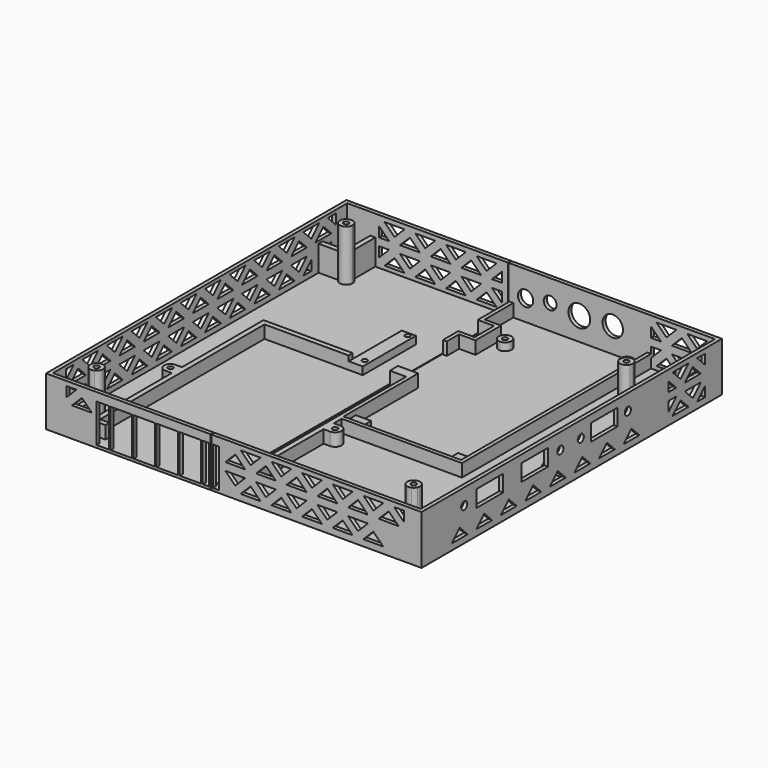
from build123d import *

# Parameters (mm, degrees)
F1_W           = 186.5100009048
F1_H           = 186.5100009048
F1_W_2         = 182.7000009048
F1_H_2         = 182.7000009048
F2_DEPTH       = 86.36
F5_W           = 186.5100009048
F5_H           = 186.5100009048
F6_DEPTH       = 1.27
F7_W           = 7.62
F7_H           = 7.62
F7_R           = 3.175
F7_R_2         = 1.27
F7_W_2         = 6.985
F7_H_2         = 33.02
F8_DEPTH       = 3.81
F9_R           = 1.27
F10_DEPTH      = 6.35
F11_R          = 5.08
F11_R_2        = 5.3975
F11_R_3        = 3.175
F11_R_4        = 3.81
F12_DEPTH      = 1.905
F13_W          = 10.668
F13_H          = 19.05
F14_DEPTH      = 2.54
F15_W          = 16.51
F15_H          = 8.255
F15_R          = 1.905
F16_DEPTH      = 1.905
F20_DEPTH      = 0.9525
F21_R          = 1.27
F22_DEPTH      = 12.7
F23_DEPTH      = 25.4
F24_W          = 8.763
F24_H          = 45.085
F24_W_2        = 11.938
F24_W_3        = 10.16
F25_DEPTH      = 25.4
F27_DEPTH      = 1.905
F29_DEPTH      = 2.54
F31_DEPTH      = 2.54
F33_DEPTH      = 2.54
F35_W          = 182.7000009048
F35_H          = 182.7000009048
F36_DEPTH      = 3.81
F37_DEPTH      = 25.4
F37_TAPER      = 45
F38_W          = 186.5100009048
F38_H          = 63.1952
F39_DEPTH      = 7.366
F41_DEPTH      = 179.1450009048
F42_W          = 5.715
F42_H          = 63.1952
F43_DEPTH      = 184.6060009048
F44_W          = 0.381
F44_H          = 186.5100009048
F45_DEPTH      = 1.271
F45_DEPTH_BACK = 25.401
F46_W          = 0.762
F46_H          = 1.905
F47_DEPTH      = 23.1648


with BuildPart() as f2:
    # F1 (on Top) → F2 (new body)
    with BuildSketch(Plane.XY):
        with Locations((78.65, -74.84)):
            Rectangle(F1_W, F1_H)
        with Locations((78.65, -74.84)):
            Rectangle(F1_W_2, F1_H_2, mode=Mode.SUBTRACT)
    extrude(amount=F2_DEPTH)

    # F5 (on Top) → F6 (join)
    with BuildSketch(Plane.XY):
        with Locations((78.65, -74.84)):
            Rectangle(F5_W, F5_H)
    extrude(amount=-F6_DEPTH)

    # F7 (on Top) → F8 (join)
    with BuildSketch(Plane.XY):
        with Locations((81.7350004524, -95.2499995476)):
            Rectangle(F7_W, F7_H)
        with Locations((132.5350004524, -95.2499995476)):
            Rectangle(F7_W, F7_H)
        with Locations((83.0050004524, -5.0799995476)):
            Circle(F7_R)
        with Locations((83.0050004524, -5.0799995476)):
            Circle(F7_R_2, mode=Mode.SUBTRACT)
        with Locations((131.2650004524, 10.1600004524)):
            Circle(F7_R)
        with Locations((131.2650004524, 10.1600004524)):
            Circle(F7_R_2, mode=Mode.SUBTRACT)
        with Locations((50.9375004524, -41.2749995476)):
            Rectangle(F7_W_2, F7_H_2)
        with Locations((51.8900004524, -53.3399995476)):
            Circle(F7_R_2, mode=Mode.SUBTRACT)
        with Locations((51.8900004524, -26.6699995476)):
            Circle(F7_R_2, mode=Mode.SUBTRACT)
    extrude(amount=F8_DEPTH)

    # F9 (on Top) → F10 (join)
    with BuildSketch(Plane.XY):
        Polygon((76.0200004524, -15.2399995476), (67.8920004524, -15.2399995476), (67.8920004524, -24.7649995476), (69.7970004524, -24.7649995476), (69.7970004524, -17.1449995476), (77.9250004524, -17.1449995476), (77.9250004524, -1.2699995476), (69.7970004524, -1.2699995476), (69.7970004524, 16.5100004524), (67.8920004524, 16.5100004524), (67.8920004524, -3.1749995476), (76.0200004524, -3.1749995476), align=None)
        with BuildLine():
            Line((136.3450004524, 16.5100004524), (136.3450004524, -99.0599995476))
            Line((136.3450004524, -99.0599995476), (77.9250004524, -99.0599995476))
            Line((77.9250004524, -99.0599995476), (77.9250004524, -52.7049995476))
            Line((77.9250004524, -52.7049995476), (67.8920004524, -52.7049995476))
            Line((67.8920004524, -52.7049995476), (67.8920004524, -57.7849995476))
            Line((67.8920004524, -57.7849995476), (76.0200004524, -57.7849995476))
            Line((76.0200004524, -57.7849995476), (76.0200004524, -100.9649995476))
            Line((76.0200004524, -100.9649995476), (76.0200004524, -159.84))
            Line((76.0200004524, -159.84), (71.3210004524, -159.84))
            Line((71.3210004524, -159.84), (71.3210004524, -162.38))
            Line((71.3210004524, -162.38), (78.5600004524, -162.38))
            Line((78.5600004524, -162.38), (78.5600004524, -112.215))
            Line((78.5600004524, -112.215), (81.7350004524, -112.215))
            ThreePointArc((81.7350004524, -112.215), (84.9100004524, -109.04), (81.7350004524, -105.865))
            Line((81.7350004524, -105.865), (78.5600004524, -105.865))
            Line((78.5600004524, -105.865), (78.5600004524, -100.9649995476))
            Line((78.5600004524, -100.9649995476), (138.2500004524, -100.9649995476))
            Line((138.2500004524, -100.9649995476), (138.2500004524, 16.5100004524))
            Line((138.2500004524, 16.5100004524), (136.3450004524, 16.5100004524))
        make_face()
        with Locations((81.7350004524, -109.04)):
            Circle(F9_R, mode=Mode.SUBTRACT)
        with BuildLine():
            Line((5.6620004524, -57.7849995476), (47.4450004524, -57.7849995476))
            Line((47.4450004524, -57.7849995476), (47.4450004524, -55.2449995476))
            Line((47.4450004524, -55.2449995476), (3.1220004524, -55.2449995476))
            Line((3.1220004524, -55.2449995476), (3.1220004524, -105.865))
            Line((3.1220004524, -105.865), (-0.0529995476, -105.865))
            ThreePointArc((-0.0529995476, -105.865), (-3.2279995476, -109.04), (-0.0529995476, -112.215))
            Line((-0.0529995476, -112.215), (3.1220004524, -112.215))
            Line((3.1220004524, -112.215), (3.1220004524, -162.38))
            Line((3.1220004524, -162.38), (10.3610004524, -162.38))
            Line((10.3610004524, -162.38), (10.3610004524, -159.84))
            Line((10.3610004524, -159.84), (5.6620004524, -159.84))
            Line((5.6620004524, -159.84), (5.6620004524, -57.7849995476))
        make_face()
        with Locations((-0.0529995476, -109.04)):
            Circle(F9_R, mode=Mode.SUBTRACT)
    extrude(amount=F10_DEPTH)

    # F11 (on face) → F12 (cut, through all)
    with BuildSketch(Plane(origin=(0, 18.4150004524, 0), x_dir=(-1, 0, 0), z_dir=(0, 1, 0))):
        with Locations((-119.2000004524, 12.319)):
            Circle(F11_R)
        with Locations((-102.5630004524, 11.43)):
            Circle(F11_R_2)
        with Locations((-88.0850004524, 12.319)):
            Circle(F11_R_3)
        with Locations((-75.8930004524, 10.414)):
            Circle(F11_R_4)
    extrude(amount=-F12_DEPTH, mode=Mode.SUBTRACT)

    # F13 (on face) → F14 (cut)
    with BuildSketch(Plane(origin=(0, -166.1900004524, 0), x_dir=(-1, 0, 0), z_dir=(0, 1, 0))):
        Polygon((-10.3610004524, 0), (-10.3610004524, 6.35), (-10.3610004524, 19.05), (-16.7110004524, 19.05), (-16.7110004524, 0), align=None)
        with Locations((-22.8070004524, 9.525)):
            Rectangle(F13_W, F13_H)
        with Locations((-34.2370004524, 9.525)):
            Rectangle(F13_W, F13_H)
        with Locations((-45.6670004524, 9.525)):
            Rectangle(F13_W, F13_H)
        with Locations((-57.0970004524, 9.525)):
            Rectangle(F13_W, F13_H)
        Polygon((-71.3210004524, 6.35), (-71.3210004524, 0), (-63.1930004524, 0), (-63.1930004524, 19.05), (-71.3210004524, 19.05), align=None)
    extrude(amount=-F14_DEPTH, mode=Mode.SUBTRACT)

    # F15 (on face) → F16 (cut, through all)
    with BuildSketch(Plane.YZ.offset(171.9050004524)):
        with Locations((-125.73, 15.24)):
            Rectangle(F15_W, F15_H)
        with Locations((-141.605, 15.24)):
            Circle(F15_R)
        with Locations((-97.79, 15.24)):
            Rectangle(F15_W, F15_H)
        with Locations((-81.915, 15.24)):
            Circle(F15_R)
        with Locations((-54.61, 15.24)):
            Rectangle(F15_W, F15_H)
        with Locations((-69.215, 15.24)):
            Circle(F15_R)
        with Locations((-40.005, 15.24)):
            Circle(F15_R)
    extrude(amount=-F16_DEPTH, mode=Mode.SUBTRACT)

    # F19 (on plane+point) → F20 (join, symmetric)
    with BuildSketch(Plane.XZ.offset(75.565)):
        Polygon((170.0000004524, 0), (170.0000004524, 21.59), (157.3000004524, 0), align=None)
    extrude(amount=F20_DEPTH, both=True)

    # F21 (on Top) → F22 (join)
    with BuildSketch(Plane.XY):
        with BuildLine():
            ThreePointArc((-1.27, 2.9099355663), (0, 3.175), (1.27, 2.9099355663))
            Line((1.27, 2.9099355663), (1.27, 16.5100004524))
            Line((1.27, 16.5100004524), (-1.27, 16.5100004524))
            Line((-1.27, 16.5100004524), (-1.27, 2.9099355663))
        make_face()
        with BuildLine():
            Line((-12.7000004524, -1.27), (-2.9099355663, -1.27))
            ThreePointArc((-2.9099355663, -1.27), (-3.175, 0), (-2.9099355663, 1.27))
            Line((-2.9099355663, 1.27), (-12.7000004524, 1.27))
            Line((-12.7000004524, 1.27), (-12.7000004524, -1.27))
        make_face()
        Circle(F21_R)
        with Locations((157.48, -22.86)):
            Circle(F21_R)
        with BuildLine():
            ThreePointArc((160.3899355663, -21.59), (160.5880275436, -22.2113168813), (160.655, -22.86))
            ThreePointArc((160.655, -22.86), (160.5880275436, -23.5086831187), (160.3899355663, -24.13))
            Line((160.3899355663, -24.13), (170.0000004524, -24.13))
            Line((170.0000004524, -24.13), (170.0000004524, -21.59))
            Line((170.0000004524, -21.59), (160.3899355663, -21.59))
        make_face()
        with Locations((157.48, -154.94)):
            Circle(F21_R)
        with BuildLine():
            ThreePointArc((160.3899355663, -153.67), (160.5880275436, -154.2913168813), (160.655, -154.94))
            ThreePointArc((160.655, -154.94), (160.5880275436, -155.5886831187), (160.3899355663, -156.21))
            Line((160.3899355663, -156.21), (170.0000004524, -156.21))
            Line((170.0000004524, -156.21), (170.0000004524, -153.67))
            Line((170.0000004524, -153.67), (160.3899355663, -153.67))
        make_face()
        with BuildLine():
            ThreePointArc((158.75, -157.8499355663), (157.48, -158.115), (156.21, -157.8499355663))
            Line((156.21, -157.8499355663), (156.21, -166.1900004524))
            Line((156.21, -166.1900004524), (158.75, -166.1900004524))
            Line((158.75, -166.1900004524), (158.75, -157.8499355663))
        make_face()
        with BuildLine():
            ThreePointArc((-2.9099355663, -156.21), (-3.175, -154.94), (-2.9099355663, -153.67))
            Line((-2.9099355663, -153.67), (-12.7000004524, -153.67))
            Line((-12.7000004524, -153.67), (-12.7000004524, -156.21))
            Line((-12.7000004524, -156.21), (-2.9099355663, -156.21))
        make_face()
        with Locations((0, -154.94)):
            Circle(F21_R)
        with BuildLine():
            Line((1.27, -166.1900004524), (1.27, -157.8499355663))
            ThreePointArc((1.27, -157.8499355663), (0, -158.115), (-1.27, -157.8499355663))
            Line((-1.27, -157.8499355663), (-1.27, -166.1900004524))
            Line((-1.27, -166.1900004524), (1.27, -166.1900004524))
        make_face()
    extrude(amount=F22_DEPTH)

    # F21 (on Top) → F23 (join)
    with BuildSketch(Plane.XY):
        with BuildLine():
            ThreePointArc((-2.9099355663, -1.27), (0.6486831187, -3.1080275436), (3.175, 0))
            ThreePointArc((3.175, 0), (2.6563955842, 1.7390191201), (1.27, 2.9099355663))
            ThreePointArc((1.27, 2.9099355663), (0, 3.175), (-1.27, 2.9099355663))
            ThreePointArc((-1.27, 2.9099355663), (-2.2450640303, 2.2450640303), (-2.9099355663, 1.27))
            ThreePointArc((-2.9099355663, 1.27), (-3.175, 0), (-2.9099355663, -1.27))
        make_face()
        Circle(F21_R, mode=Mode.SUBTRACT)
        with BuildLine():
            ThreePointArc((160.3899355663, -24.13), (160.5880275436, -23.5086831187), (160.655, -22.86))
            ThreePointArc((160.655, -22.86), (160.5880275436, -22.2113168813), (160.3899355663, -21.59))
            ThreePointArc((160.3899355663, -21.59), (154.305, -22.86), (160.3899355663, -24.13))
        make_face()
        with Locations((157.48, -22.86)):
            Circle(F21_R, mode=Mode.SUBTRACT)
        with BuildLine():
            ThreePointArc((1.27, -157.8499355663), (2.6563955842, -156.6790191201), (3.175, -154.94))
            ThreePointArc((3.175, -154.94), (0.6486831187, -151.8319724564), (-2.9099355663, -153.67))
            ThreePointArc((-2.9099355663, -153.67), (-3.175, -154.94), (-2.9099355663, -156.21))
            ThreePointArc((-2.9099355663, -156.21), (-2.2450640303, -157.1850640303), (-1.27, -157.8499355663))
            ThreePointArc((-1.27, -157.8499355663), (0, -158.115), (1.27, -157.8499355663))
        make_face()
        with Locations((0, -154.94)):
            Circle(F21_R, mode=Mode.SUBTRACT)
        with BuildLine():
            ThreePointArc((160.3899355663, -156.21), (160.5880275436, -155.5886831187), (160.655, -154.94))
            ThreePointArc((160.655, -154.94), (160.5880275436, -154.2913168813), (160.3899355663, -153.67))
            ThreePointArc((160.3899355663, -153.67), (155.2349359697, -152.6949359697), (156.21, -157.8499355663))
            ThreePointArc((156.21, -157.8499355663), (157.48, -158.115), (158.75, -157.8499355663))
            ThreePointArc((158.75, -157.8499355663), (159.7250640303, -157.1850640303), (160.3899355663, -156.21))
        make_face()
        with Locations((157.48, -154.94)):
            Circle(F21_R, mode=Mode.SUBTRACT)
    extrude(amount=F23_DEPTH)

    # F24 (on Front) → F25 (cut)
    with BuildSketch(Plane.XZ):
        with Locations((11.8999, 45.7073)):
            Rectangle(F24_W, F24_H)
        with Locations((23.0124, 45.7073)):
            Rectangle(F24_W_2, F24_H)
        with Locations((35.7124, 45.7073)):
            Rectangle(F24_W_2, F24_H)
        with Locations((48.4124, 45.7073)):
            Rectangle(F24_W_2, F24_H)
        with Locations((61.1124, 45.7073)):
            Rectangle(F24_W_2, F24_H)
        with Locations((73.8124, 45.7073)):
            Rectangle(F24_W_2, F24_H)
        with Locations((86.5124, 45.7073)):
            Rectangle(F24_W_2, F24_H)
        with Locations((99.2124, 45.7073)):
            Rectangle(F24_W_2, F24_H)
        with Locations((111.9124, 45.7073)):
            Rectangle(F24_W_2, F24_H)
        with Locations((124.6124, 45.7073)):
            Rectangle(F24_W_2, F24_H)
        with Locations((137.3124, 45.7073)):
            Rectangle(F24_W_2, F24_H)
        with Locations((150.0124, 45.7073)):
            Rectangle(F24_W_2, F24_H)
        with Locations((161.8234, 45.7073)):
            Rectangle(F24_W_3, F24_H)
    extrude(amount=-F25_DEPTH, mode=Mode.SUBTRACT)

    # F26 (on face) → F27 (cut, through all)
    with BuildSketch(Plane.XZ.offset(-16.5100004524)):
        Polygon((23.3409231637, 9.525), (18.415, 9.525), (13.4890768363, 9.525), (18.415, 4.5990768363), align=None)
        Polygon((15.7209231637, 1.905), (10.795, 6.8309231637), (5.8690768363, 1.905), align=None)
        Polygon((3.175, 9.525), (3.175, 4.5990768363), (8.1009231637, 9.525), align=None)
        Polygon((33.655, 9.525), (28.7290768363, 9.525), (33.655, 4.5990768363), (38.5809231637, 9.525), align=None)
        Polygon((21.1090768363, 1.905), (30.9609231637, 1.905), (26.035, 6.8309231637), align=None)
        Polygon((41.275, 6.8309231637), (36.3490768363, 1.905), (46.2009231637, 1.905), align=None)
        Polygon((48.895, 9.525), (43.9690768363, 9.525), (48.895, 4.5990768363), (53.8209231637, 9.525), align=None)
        Polygon((8.1009231637, 13.335), (3.175, 18.2609231637), (3.175, 13.335), align=None)
        Polygon((15.7209231637, 20.955), (5.8690768363, 20.955), (10.795, 16.0290768363), align=None)
        Polygon((18.415, 18.2609231637), (13.4890768363, 13.335), (18.415, 13.335), (23.3409231637, 13.335), align=None)
        Polygon((21.1090768363, 20.955), (26.035, 16.0290768363), (30.9609231637, 20.955), align=None)
        Polygon((38.5809231637, 13.335), (33.655, 18.2609231637), (28.7290768363, 13.335), (33.655, 13.335), align=None)
        Polygon((36.3490768363, 20.955), (41.275, 16.0290768363), (46.2009231637, 20.955), align=None)
        Polygon((48.895, 18.2609231637), (43.9690768363, 13.335), (48.895, 13.335), (53.8209231637, 13.335), align=None)
        Polygon((51.5890768363, 20.955), (56.515, 16.0290768363), (61.4409231637, 20.955), align=None)
        Polygon((64.135, 13.335), (64.135, 18.2609231637), (59.2090768363, 13.335), align=None)
        Polygon((64.135, 9.525), (59.2090768363, 9.525), (64.135, 4.5990768363), align=None)
        Polygon((61.4409231637, 1.905), (56.515, 6.8309231637), (51.5890768363, 1.905), align=None)
        Polygon((138.2500004524, 9.525), (138.2500004524, 4.5990768363), (143.1759236161, 9.525), align=None)
        Polygon((140.9440772887, 20.955), (145.8700004524, 16.0290768363), (150.7959236161, 20.955), align=None)
        Polygon((143.1759236161, 13.335), (138.2500004524, 18.2609231637), (138.2500004524, 13.335), align=None)
        Polygon((168.7300004524, 13.335), (168.7300004524, 18.2609231637), (163.8040772887, 13.335), align=None)
        Polygon((158.4159236161, 9.525), (153.4900004524, 9.525), (148.5640772887, 9.525), (153.4900004524, 4.5990768363), align=None)
        Polygon((148.5640772887, 13.335), (153.4900004524, 13.335), (158.4159236161, 13.335), (153.4900004524, 18.2609231637), align=None)
        Polygon((168.7300004524, 9.525), (163.8040772887, 9.525), (168.7300004524, 4.5990768363), align=None)
        Polygon((161.1100004524, 20.955), (161.1100004524, 16.0290768363), (166.0359236161, 20.955), align=None)
        Polygon((156.1840772887, 20.955), (161.1100004524, 16.0290768363), (161.1100004524, 20.955), align=None)
        Polygon((161.1100004524, 1.905), (161.1100004524, 6.8309231637), (156.1840772887, 1.905), align=None)
        Polygon((166.0359236161, 1.905), (161.1100004524, 6.8309231637), (161.1100004524, 1.905), align=None)
        Polygon((150.7959236161, 1.905), (145.8700004524, 6.8309231637), (140.9440772887, 1.905), align=None)
    extrude(amount=-F27_DEPTH, mode=Mode.SUBTRACT)

    # F28 (on face) → F29 (cut)
    with BuildSketch(Plane.XZ.offset(168.0950004524)):
        Polygon((8.1009231637, 13.335), (3.175, 18.2609231637), (-1.7509231637, 13.335), (3.175, 13.335), align=None)
        Polygon((-4.445, 16.0290768363), (0.4809231637, 20.955), (-4.445, 20.955), align=None)
        Polygon((8.1009231637, 36.195), (3.175, 41.1209231637), (-1.7509231637, 36.195), (3.175, 36.195), align=None)
        Polygon((3.175, 32.385), (-1.7509231637, 32.385), (3.175, 27.4590768363), (8.1009231637, 32.385), align=None)
        Polygon((10.795, 29.6909231637), (5.8690768363, 24.765), (15.7209231637, 24.765), align=None)
        Polygon((15.7209231637, 43.815), (5.8690768363, 43.815), (10.795, 38.8890768363), align=None)
        Polygon((8.1009231637, 59.055), (3.175, 63.9809231637), (-1.7509231637, 59.055), (3.175, 59.055), align=None)
        Polygon((3.175, 55.245), (-1.7509231637, 55.245), (3.175, 50.3190768363), (8.1009231637, 55.245), align=None)
        Polygon((10.795, 52.5509231637), (5.8690768363, 47.625), (15.7209231637, 47.625), align=None)
        Polygon((15.7209231637, 66.675), (5.8690768363, 66.675), (10.795, 61.7490768363), align=None)
        Polygon((23.3409231637, 36.195), (18.415, 41.1209231637), (13.4890768363, 36.195), (18.415, 36.195), align=None)
        Polygon((18.415, 32.385), (13.4890768363, 32.385), (18.415, 27.4590768363), (23.3409231637, 32.385), align=None)
        Polygon((26.035, 29.6909231637), (21.1090768363, 24.765), (30.9609231637, 24.765), align=None)
        Polygon((30.9609231637, 43.815), (21.1090768363, 43.815), (26.035, 38.8890768363), align=None)
        Polygon((23.3409231637, 59.055), (18.415, 63.9809231637), (13.4890768363, 59.055), (18.415, 59.055), align=None)
        Polygon((18.415, 55.245), (13.4890768363, 55.245), (18.415, 50.3190768363), (23.3409231637, 55.245), align=None)
        Polygon((26.035, 52.5509231637), (21.1090768363, 47.625), (30.9609231637, 47.625), align=None)
        Polygon((30.9609231637, 66.675), (21.1090768363, 66.675), (26.035, 61.7490768363), align=None)
        Polygon((38.5809231637, 36.195), (33.655, 41.1209231637), (28.7290768363, 36.195), (33.655, 36.195), align=None)
        Polygon((33.655, 32.385), (28.7290768363, 32.385), (33.655, 27.4590768363), (38.5809231637, 32.385), align=None)
        Polygon((41.275, 29.6909231637), (36.3490768363, 24.765), (46.2009231637, 24.765), align=None)
        Polygon((46.2009231637, 43.815), (36.3490768363, 43.815), (41.275, 38.8890768363), align=None)
        Polygon((38.5809231637, 59.055), (33.655, 63.9809231637), (28.7290768363, 59.055), (33.655, 59.055), align=None)
        Polygon((33.655, 55.245), (28.7290768363, 55.245), (33.655, 50.3190768363), (38.5809231637, 55.245), align=None)
        Polygon((41.275, 52.5509231637), (36.3490768363, 47.625), (46.2009231637, 47.625), align=None)
        Polygon((46.2009231637, 66.675), (36.3490768363, 66.675), (41.275, 61.7490768363), align=None)
        Polygon((53.8209231637, 36.195), (48.895, 41.1209231637), (43.9690768363, 36.195), (48.895, 36.195), align=None)
        Polygon((48.895, 32.385), (43.9690768363, 32.385), (48.895, 27.4590768363), (53.8209231637, 32.385), align=None)
        Polygon((56.515, 29.6909231637), (51.5890768363, 24.765), (61.4409231637, 24.765), align=None)
        Polygon((61.4409231637, 43.815), (51.5890768363, 43.815), (56.515, 38.8890768363), align=None)
        Polygon((53.8209231637, 59.055), (48.895, 63.9809231637), (43.9690768363, 59.055), (48.895, 59.055), align=None)
        Polygon((48.895, 55.245), (43.9690768363, 55.245), (48.895, 50.3190768363), (53.8209231637, 55.245), align=None)
        Polygon((56.515, 52.5509231637), (51.5890768363, 47.625), (61.4409231637, 47.625), align=None)
        Polygon((61.4409231637, 66.675), (51.5890768363, 66.675), (56.515, 61.7490768363), align=None)
        Polygon((69.0609231637, 36.195), (64.135, 41.1209231637), (59.2090768363, 36.195), (64.135, 36.195), align=None)
        Polygon((64.135, 32.385), (59.2090768363, 32.385), (64.135, 27.4590768363), (69.0609231637, 32.385), align=None)
        Polygon((71.755, 29.6909231637), (66.8290768363, 24.765), (76.6809231637, 24.765), align=None)
        Polygon((76.6809231637, 43.815), (66.8290768363, 43.815), (71.755, 38.8890768363), align=None)
        Polygon((69.0609231637, 59.055), (64.135, 63.9809231637), (59.2090768363, 59.055), (64.135, 59.055), align=None)
        Polygon((64.135, 55.245), (59.2090768363, 55.245), (64.135, 50.3190768363), (69.0609231637, 55.245), align=None)
        Polygon((71.755, 52.5509231637), (66.8290768363, 47.625), (76.6809231637, 47.625), align=None)
        Polygon((76.6809231637, 66.675), (66.8290768363, 66.675), (71.755, 61.7490768363), align=None)
        Polygon((84.3009231637, 13.335), (79.375, 18.2609231637), (74.4490768363, 13.335), (79.375, 13.335), align=None)
        Polygon((79.375, 9.525), (74.4490768363, 9.525), (79.375, 4.5990768363), (84.3009231637, 9.525), align=None)
        Polygon((86.995, 6.8309231637), (82.0690768363, 1.905), (91.9209231637, 1.905), align=None)
        Polygon((91.9209231637, 20.955), (82.0690768363, 20.955), (86.995, 16.0290768363), align=None)
        Polygon((84.3009231637, 36.195), (79.375, 41.1209231637), (74.4490768363, 36.195), (79.375, 36.195), align=None)
        Polygon((79.375, 32.385), (74.4490768363, 32.385), (79.375, 27.4590768363), (84.3009231637, 32.385), align=None)
        Polygon((86.995, 29.6909231637), (82.0690768363, 24.765), (91.9209231637, 24.765), align=None)
        Polygon((91.9209231637, 43.815), (82.0690768363, 43.815), (86.995, 38.8890768363), align=None)
        Polygon((84.3009231637, 59.055), (79.375, 63.9809231637), (74.4490768363, 59.055), (79.375, 59.055), align=None)
        Polygon((79.375, 55.245), (74.4490768363, 55.245), (79.375, 50.3190768363), (84.3009231637, 55.245), align=None)
        Polygon((86.995, 52.5509231637), (82.0690768363, 47.625), (91.9209231637, 47.625), align=None)
        Polygon((91.9209231637, 66.675), (82.0690768363, 66.675), (86.995, 61.7490768363), align=None)
        Polygon((99.5409231637, 13.335), (94.615, 18.2609231637), (89.6890768363, 13.335), (94.615, 13.335), align=None)
        Polygon((94.615, 9.525), (89.6890768363, 9.525), (94.615, 4.5990768363), (99.5409231637, 9.525), align=None)
        Polygon((102.235, 6.8309231637), (97.3090768363, 1.905), (107.1609231637, 1.905), align=None)
        Polygon((107.1609231637, 20.955), (97.3090768363, 20.955), (102.235, 16.0290768363), align=None)
        Polygon((99.5409231637, 36.195), (94.615, 41.1209231637), (89.6890768363, 36.195), (94.615, 36.195), align=None)
        Polygon((94.615, 32.385), (89.6890768363, 32.385), (94.615, 27.4590768363), (99.5409231637, 32.385), align=None)
        Polygon((102.235, 29.6909231637), (97.3090768363, 24.765), (107.1609231637, 24.765), align=None)
        Polygon((107.1609231637, 43.815), (97.3090768363, 43.815), (102.235, 38.8890768363), align=None)
        Polygon((99.5409231637, 59.055), (94.615, 63.9809231637), (89.6890768363, 59.055), (94.615, 59.055), align=None)
        Polygon((94.615, 55.245), (89.6890768363, 55.245), (94.615, 50.3190768363), (99.5409231637, 55.245), align=None)
        Polygon((102.235, 52.5509231637), (97.3090768363, 47.625), (107.1609231637, 47.625), align=None)
        Polygon((107.1609231637, 66.675), (97.3090768363, 66.675), (102.235, 61.7490768363), align=None)
        Polygon((114.7809231637, 13.335), (109.855, 18.2609231637), (104.9290768363, 13.335), (109.855, 13.335), align=None)
        Polygon((109.855, 9.525), (104.9290768363, 9.525), (109.855, 4.5990768363), (114.7809231637, 9.525), align=None)
        Polygon((117.475, 6.8309231637), (112.5490768363, 1.905), (122.4009231637, 1.905), align=None)
        Polygon((122.4009231637, 20.955), (112.5490768363, 20.955), (117.475, 16.0290768363), align=None)
        Polygon((114.7809231637, 36.195), (109.855, 41.1209231637), (104.9290768363, 36.195), (109.855, 36.195), align=None)
        Polygon((109.855, 32.385), (104.9290768363, 32.385), (109.855, 27.4590768363), (114.7809231637, 32.385), align=None)
        Polygon((117.475, 29.6909231637), (112.5490768363, 24.765), (122.4009231637, 24.765), align=None)
        Polygon((122.4009231637, 43.815), (112.5490768363, 43.815), (117.475, 38.8890768363), align=None)
        Polygon((114.7809231637, 59.055), (109.855, 63.9809231637), (104.9290768363, 59.055), (109.855, 59.055), align=None)
        Polygon((109.855, 55.245), (104.9290768363, 55.245), (109.855, 50.3190768363), (114.7809231637, 55.245), align=None)
        Polygon((117.475, 52.5509231637), (112.5490768363, 47.625), (122.4009231637, 47.625), align=None)
        Polygon((122.4009231637, 66.675), (112.5490768363, 66.675), (117.475, 61.7490768363), align=None)
        Polygon((130.0209231637, 13.335), (125.095, 18.2609231637), (120.1690768363, 13.335), (125.095, 13.335), align=None)
        Polygon((125.095, 9.525), (120.1690768363, 9.525), (125.095, 4.5990768363), (130.0209231637, 9.525), align=None)
        Polygon((132.715, 6.8309231637), (127.7890768363, 1.905), (137.6409231637, 1.905), align=None)
        Polygon((137.6409231637, 20.955), (127.7890768363, 20.955), (132.715, 16.0290768363), align=None)
        Polygon((130.0209231637, 36.195), (125.095, 41.1209231637), (120.1690768363, 36.195), (125.095, 36.195), align=None)
        Polygon((125.095, 32.385), (120.1690768363, 32.385), (125.095, 27.4590768363), (130.0209231637, 32.385), align=None)
        Polygon((132.715, 29.6909231637), (127.7890768363, 24.765), (137.6409231637, 24.765), align=None)
        Polygon((137.6409231637, 43.815), (127.7890768363, 43.815), (132.715, 38.8890768363), align=None)
        Polygon((130.0209231637, 59.055), (125.095, 63.9809231637), (120.1690768363, 59.055), (125.095, 59.055), align=None)
        Polygon((125.095, 55.245), (120.1690768363, 55.245), (125.095, 50.3190768363), (130.0209231637, 55.245), align=None)
        Polygon((132.715, 52.5509231637), (127.7890768363, 47.625), (137.6409231637, 47.625), align=None)
        Polygon((137.6409231637, 66.675), (127.7890768363, 66.675), (132.715, 61.7490768363), align=None)
        Polygon((145.2609231637, 13.335), (140.335, 18.2609231637), (135.4090768363, 13.335), (140.335, 13.335), align=None)
        Polygon((140.335, 9.525), (135.4090768363, 9.525), (140.335, 4.5990768363), (145.2609231637, 9.525), align=None)
        Polygon((147.955, 6.8309231637), (143.0290768363, 1.905), (152.8809231637, 1.905), align=None)
        Polygon((152.8809231637, 20.955), (143.0290768363, 20.955), (147.955, 16.0290768363), align=None)
        Polygon((145.2609231637, 36.195), (140.335, 41.1209231637), (135.4090768363, 36.195), (140.335, 36.195), align=None)
        Polygon((140.335, 32.385), (135.4090768363, 32.385), (140.335, 27.4590768363), (145.2609231637, 32.385), align=None)
        Polygon((147.955, 29.6909231637), (143.0290768363, 24.765), (152.8809231637, 24.765), align=None)
        Polygon((152.8809231637, 43.815), (143.0290768363, 43.815), (147.955, 38.8890768363), align=None)
        Polygon((145.2609231637, 59.055), (140.335, 63.9809231637), (135.4090768363, 59.055), (140.335, 59.055), align=None)
        Polygon((140.335, 55.245), (135.4090768363, 55.245), (140.335, 50.3190768363), (145.2609231637, 55.245), align=None)
        Polygon((147.955, 52.5509231637), (143.0290768363, 47.625), (152.8809231637, 47.625), align=None)
        Polygon((152.8809231637, 66.675), (143.0290768363, 66.675), (147.955, 61.7490768363), align=None)
        Polygon((160.5009231637, 13.335), (155.575, 18.2609231637), (150.6490768363, 13.335), (155.575, 13.335), align=None)
        Polygon((163.195, 20.955), (158.2690768363, 20.955), (163.195, 16.0290768363), align=None)
        Polygon((160.5009231637, 36.195), (155.575, 41.1209231637), (150.6490768363, 36.195), (155.575, 36.195), align=None)
        Polygon((155.575, 32.385), (150.6490768363, 32.385), (155.575, 27.4590768363), (160.5009231637, 32.385), align=None)
        Polygon((163.195, 29.6909231637), (158.2690768363, 24.765), (163.195, 24.765), align=None)
        Polygon((163.195, 43.815), (158.2690768363, 43.815), (163.195, 38.8890768363), align=None)
        Polygon((160.5009231637, 59.055), (155.575, 63.9809231637), (150.6490768363, 59.055), (155.575, 59.055), align=None)
        Polygon((155.575, 55.245), (150.6490768363, 55.245), (155.575, 50.3190768363), (160.5009231637, 55.245), align=None)
        Polygon((163.195, 52.5509231637), (158.2690768363, 47.625), (163.195, 47.625), align=None)
        Polygon((163.195, 66.675), (158.2690768363, 66.675), (163.195, 61.7490768363), align=None)
        Polygon((-4.445, 43.815), (-4.445, 38.8890768363), (0.4809231637, 43.815), align=None)
        Polygon((0.4809231637, 24.765), (-4.445, 29.6909231637), (-4.445, 24.765), align=None)
        Polygon((-4.445, 66.675), (-4.445, 61.7490768363), (0.4809231637, 66.675), align=None)
        Polygon((0.4809231637, 47.625), (-4.445, 52.5509231637), (-4.445, 47.625), align=None)
    extrude(amount=-F29_DEPTH, mode=Mode.SUBTRACT)

    # F30 (on face) → F31 (cut)
    with BuildSketch(Plane.YZ.offset(171.9050004524)):
        Polygon((-147.1091767458, 58.98052284), (-152.0350999095, 63.9064460037), (-156.9610230731, 58.98052284), align=None)
        Polygon((-147.1091767458, 55.17052284), (-156.9610230731, 55.17052284), (-152.0350999095, 50.2445996763), align=None)
        Polygon((-144.4150999095, 52.4764460037), (-149.3410230731, 47.55052284), (-139.4891767458, 47.55052284), align=None)
        Polygon((-139.4891767458, 66.60052284), (-149.3410230731, 66.60052284), (-144.4150999095, 61.6745996763), align=None)
        Polygon((-131.8691767458, 58.98052284), (-136.7950999095, 63.9064460037), (-141.7210230731, 58.98052284), align=None)
        Polygon((-131.8691767458, 55.17052284), (-141.7210230731, 55.17052284), (-136.7950999095, 50.2445996763), align=None)
        Polygon((-129.1750999095, 52.4764460037), (-134.1010230731, 47.55052284), (-124.2491767458, 47.55052284), align=None)
        Polygon((-124.2491767458, 66.60052284), (-134.1010230731, 66.60052284), (-129.1750999095, 61.6745996763), align=None)
        Polygon((-116.6291767458, 58.98052284), (-121.5550999095, 63.9064460037), (-126.4810230731, 58.98052284), align=None)
        Polygon((-116.6291767458, 55.17052284), (-126.4810230731, 55.17052284), (-121.5550999095, 50.2445996763), align=None)
        Polygon((-113.9350999095, 52.4764460037), (-118.8610230731, 47.55052284), (-109.0091767458, 47.55052284), align=None)
        Polygon((-109.0091767458, 66.60052284), (-118.8610230731, 66.60052284), (-113.9350999095, 61.6745996763), align=None)
        Polygon((-101.3891767458, 58.98052284), (-106.3150999095, 63.9064460037), (-111.2410230731, 58.98052284), align=None)
        Polygon((-101.3891767458, 55.17052284), (-111.2410230731, 55.17052284), (-106.3150999095, 50.2445996763), align=None)
        Polygon((-98.6950999095, 52.4764460037), (-103.6210230731, 47.55052284), (-93.7691767458, 47.55052284), align=None)
        Polygon((-93.7691767458, 66.60052284), (-103.6210230731, 66.60052284), (-98.6950999095, 61.6745996763), align=None)
        Polygon((-86.1491767458, 58.98052284), (-91.0750999095, 63.9064460037), (-96.0010230731, 58.98052284), align=None)
        Polygon((-86.1491767458, 55.17052284), (-96.0010230731, 55.17052284), (-91.0750999095, 50.2445996763), align=None)
        Polygon((-83.4550999095, 52.4764460037), (-88.3810230731, 47.55052284), (-78.5291767458, 47.55052284), align=None)
        Polygon((-78.5291767458, 66.60052284), (-88.3810230731, 66.60052284), (-83.4550999095, 61.6745996763), align=None)
        Polygon((-70.9091767458, 58.98052284), (-75.8350999095, 63.9064460037), (-80.7610230731, 58.98052284), align=None)
        Polygon((-70.9091767458, 55.17052284), (-80.7610230731, 55.17052284), (-75.8350999095, 50.2445996763), align=None)
        Polygon((-68.2150999095, 52.4764460037), (-73.1410230731, 47.55052284), (-63.2891767458, 47.55052284), align=None)
        Polygon((-63.2891767458, 66.60052284), (-73.1410230731, 66.60052284), (-68.2150999095, 61.6745996763), align=None)
        Polygon((-55.6691767458, 58.98052284), (-60.5950999095, 63.9064460037), (-65.5210230731, 58.98052284), align=None)
        Polygon((-55.6691767458, 55.17052284), (-65.5210230731, 55.17052284), (-60.5950999095, 50.2445996763), align=None)
        Polygon((-52.9750999095, 52.4764460037), (-57.9010230731, 47.55052284), (-48.0491767458, 47.55052284), align=None)
        Polygon((-48.0491767458, 66.60052284), (-57.9010230731, 66.60052284), (-52.9750999095, 61.6745996763), align=None)
        Polygon((-40.4291767458, 58.98052284), (-45.3550999095, 63.9064460037), (-50.2810230731, 58.98052284), align=None)
        Polygon((-40.4291767458, 55.17052284), (-50.2810230731, 55.17052284), (-45.3550999095, 50.2445996763), align=None)
        Polygon((-37.7350999095, 52.4764460037), (-42.6610230731, 47.55052284), (-32.8091767458, 47.55052284), align=None)
        Polygon((-32.8091767458, 66.60052284), (-42.6610230731, 66.60052284), (-37.7350999095, 61.6745996763), align=None)
        Polygon((-25.1891767458, 58.98052284), (-30.1150999095, 63.9064460037), (-35.0410230731, 58.98052284), align=None)
        Polygon((-25.1891767458, 55.17052284), (-35.0410230731, 55.17052284), (-30.1150999095, 50.2445996763), align=None)
        Polygon((-22.4950999095, 52.4764460037), (-27.4210230731, 47.55052284), (-17.5691767458, 47.55052284), align=None)
        Polygon((-17.5691767458, 66.60052284), (-27.4210230731, 66.60052284), (-22.4950999095, 61.6745996763), align=None)
        Polygon((-9.9491767458, 58.98052284), (-14.8750999095, 63.9064460037), (-19.8010230731, 58.98052284), align=None)
        Polygon((-9.9491767458, 55.17052284), (-19.8010230731, 55.17052284), (-14.8750999095, 50.2445996763), align=None)
        Polygon((-7.2550999095, 52.4764460037), (-12.1810230731, 47.55052284), (-2.3291767458, 47.55052284), align=None)
        Polygon((-2.3291767458, 66.60052284), (-12.1810230731, 66.60052284), (-7.2550999095, 61.6745996763), align=None)
        Polygon((5.2908232542, 58.98052284), (0.3649000905, 63.9064460037), (-4.5610230731, 58.98052284), align=None)
        Polygon((5.2908232542, 55.17052284), (-4.5610230731, 55.17052284), (0.3649000905, 50.2445996763), align=None)
        Polygon((7.9849000905, 52.4764460037), (3.0589769269, 47.55052284), (7.9849000905, 47.55052284), align=None)
        Polygon((7.9849000905, 66.60052284), (3.0589769269, 66.60052284), (7.9849000905, 61.6745996763), align=None)
        Polygon((-159.6550999095, 66.60052284), (-159.6550999095, 61.6745996763), (-154.7291767458, 66.60052284), align=None)
        Polygon((-154.7291767458, 47.55052284), (-159.6550999095, 52.4764460037), (-159.6550999095, 47.55052284), align=None)
        Polygon((-121.5550999095, 41.0464460037), (-126.4810230731, 36.12052284), (-116.6291767458, 36.12052284), align=None)
        Polygon((-109.0091767458, 24.69052284), (-113.9350999095, 29.6164460037), (-118.8610230731, 24.69052284), align=None)
        Polygon((7.9849000905, 43.74052284), (3.0589769269, 43.74052284), (7.9849000905, 38.8145996763), align=None)
        Polygon((-126.4810230731, 32.31052284), (-121.5550999095, 27.3845996763), (-116.6291767458, 32.31052284), align=None)
        Polygon((-63.2891767458, 43.74052284), (-73.1410230731, 43.74052284), (-68.2150999095, 38.8145996763), align=None)
        Polygon((-98.6950999095, 29.6164460037), (-103.6210230731, 24.69052284), (-93.7691767458, 24.69052284), align=None)
        Polygon((-35.0410230731, 32.31052284), (-30.1150999095, 27.3845996763), (-25.1891767458, 32.31052284), align=None)
        Polygon((-32.8091767458, 43.74052284), (-42.6610230731, 43.74052284), (-37.7350999095, 38.8145996763), align=None)
        Polygon((-124.2491767458, 24.69052284), (-129.1750999095, 29.6164460037), (-134.1010230731, 24.69052284), align=None)
        Polygon((-4.5610230731, 32.31052284), (0.3649000905, 27.3845996763), (5.2908232542, 32.31052284), align=None)
        Polygon((-48.0491767458, 43.74052284), (-57.9010230731, 43.74052284), (-52.9750999095, 38.8145996763), align=None)
        Polygon((-19.8010230731, 32.31052284), (-14.8750999095, 27.3845996763), (-9.9491767458, 32.31052284), align=None)
        Polygon((-78.5291767458, 43.74052284), (-88.3810230731, 43.74052284), (-83.4550999095, 38.8145996763), align=None)
        Polygon((-101.3891767458, 36.12052284), (-106.3150999095, 41.0464460037), (-111.2410230731, 36.12052284), align=None)
        Polygon((-55.6691767458, 36.12052284), (-60.5950999095, 41.0464460037), (-65.5210230731, 36.12052284), align=None)
        Polygon((-152.0350999095, 41.0464460037), (-156.9610230731, 36.12052284), (-147.1091767458, 36.12052284), align=None)
        Polygon((-147.1091767458, 32.31052284), (-156.9610230731, 32.31052284), (-152.0350999095, 27.3845996763), align=None)
        Polygon((-139.4891767458, 24.69052284), (-144.4150999095, 29.6164460037), (-149.3410230731, 24.69052284), align=None)
        Polygon((-50.2810230731, 32.31052284), (-45.3550999095, 27.3845996763), (-40.4291767458, 32.31052284), align=None)
        Polygon((-124.2491767458, 43.74052284), (-134.1010230731, 43.74052284), (-129.1750999095, 38.8145996763), align=None)
        Polygon((-40.4291767458, 36.12052284), (-45.3550999095, 41.0464460037), (-50.2810230731, 36.12052284), align=None)
        Polygon((-111.2410230731, 32.31052284), (-106.3150999095, 27.3845996763), (-101.3891767458, 32.31052284), align=None)
        Polygon((-30.1150999095, 41.0464460037), (-35.0410230731, 36.12052284), (-25.1891767458, 36.12052284), align=None)
        Polygon((-27.4210230731, 43.74052284), (-22.4950999095, 38.8145996763), (-17.5691767458, 43.74052284), align=None)
        Polygon((-65.5210230731, 32.31052284), (-60.5950999095, 27.3845996763), (-55.6691767458, 32.31052284), align=None)
        Polygon((-14.8750999095, 41.0464460037), (-19.8010230731, 36.12052284), (-9.9491767458, 36.12052284), align=None)
        Polygon((-96.0010230731, 32.31052284), (-91.0750999095, 27.3845996763), (-86.1491767458, 32.31052284), align=None)
        Polygon((-93.7691767458, 43.74052284), (-103.6210230731, 43.74052284), (-98.6950999095, 38.8145996763), align=None)
        Polygon((-70.9091767458, 36.12052284), (-75.8350999095, 41.0464460037), (-80.7610230731, 36.12052284), align=None)
        Polygon((5.2908232542, 36.12052284), (0.3649000905, 41.0464460037), (-4.5610230731, 36.12052284), align=None)
        Polygon((-22.4950999095, 29.6164460037), (-27.4210230731, 24.69052284), (-17.5691767458, 24.69052284), align=None)
        Polygon((-48.0491767458, 24.69052284), (-52.9750999095, 29.6164460037), (-57.9010230731, 24.69052284), align=None)
        Polygon((-70.9091767458, 32.31052284), (-80.7610230731, 32.31052284), (-75.8350999095, 27.3845996763), align=None)
        Polygon((-7.2550999095, 29.6164460037), (-12.1810230731, 24.69052284), (-2.3291767458, 24.69052284), align=None)
        Polygon((-139.4891767458, 43.74052284), (-149.3410230731, 43.74052284), (-144.4150999095, 38.8145996763), align=None)
        Polygon((-2.3291767458, 43.74052284), (-12.1810230731, 43.74052284), (-7.2550999095, 38.8145996763), align=None)
        Polygon((-91.0750999095, 41.0464460037), (-96.0010230731, 36.12052284), (-86.1491767458, 36.12052284), align=None)
        Polygon((-37.7350999095, 29.6164460037), (-42.6610230731, 24.69052284), (-32.8091767458, 24.69052284), align=None)
        Polygon((-68.2150999095, 29.6164460037), (-73.1410230731, 24.69052284), (-63.2891767458, 24.69052284), align=None)
        Polygon((-78.5291767458, 24.69052284), (-83.4550999095, 29.6164460037), (-88.3810230731, 24.69052284), align=None)
        Polygon((7.9849000905, 29.6164460037), (3.0589769269, 24.69052284), (7.9849000905, 24.69052284), align=None)
        Polygon((-109.0091767458, 43.74052284), (-118.8610230731, 43.74052284), (-113.9350999095, 38.8145996763), align=None)
        Polygon((-131.8691767458, 36.12052284), (-136.7950999095, 41.0464460037), (-141.7210230731, 36.12052284), align=None)
        Polygon((-159.6550999095, 38.8145996763), (-154.7291767458, 43.74052284), (-159.6550999095, 43.74052284), align=None)
        Polygon((-131.8691767458, 32.31052284), (-141.7210230731, 32.31052284), (-136.7950999095, 27.3845996763), align=None)
        Polygon((-154.7291767458, 24.69052284), (-159.6550999095, 29.6164460037), (-159.6550999095, 24.69052284), align=None)
        Polygon((-109.0091767458, 1.83052284), (-113.9350999095, 6.7564460037), (-118.8610230731, 1.83052284), align=None)
        Polygon((7.9849000905, 20.88052284), (3.0589769269, 20.88052284), (7.9849000905, 15.9545996763), align=None)
        Polygon((-98.6950999095, 6.7564460037), (-103.6210230731, 1.83052284), (-93.7691767458, 1.83052284), align=None)
        Polygon((-124.2491767458, 1.83052284), (-129.1750999095, 6.7564460037), (-134.1010230731, 1.83052284), align=None)
        Polygon((-4.5610230731, 9.45052284), (0.3649000905, 4.5245996763), (5.2908232542, 9.45052284), align=None)
        Polygon((-14.8750999095, 9.45052284), (-14.8750999095, 4.5245996763), (-9.9491767458, 9.45052284), align=None)
        Polygon((-139.4891767458, 1.83052284), (-144.4150999095, 6.7564460037), (-149.3410230731, 1.83052284), align=None)
        Polygon((-14.8750999095, 18.1864460037), (-14.8750999095, 13.26052284), (-9.9491767458, 13.26052284), align=None)
        Polygon((5.2908232542, 13.26052284), (0.3649000905, 18.1864460037), (-4.5610230731, 13.26052284), align=None)
        Polygon((-48.0491767458, 1.83052284), (-52.9750999095, 6.7564460037), (-57.9010230731, 1.83052284), align=None)
        Polygon((-7.2550999095, 6.7564460037), (-12.1810230731, 1.83052284), (-2.3291767458, 1.83052284), align=None)
        Polygon((-2.3291767458, 20.88052284), (-12.1810230731, 20.88052284), (-7.2550999095, 15.9545996763), align=None)
        Polygon((-37.7350999095, 6.7564460037), (-42.6610230731, 1.83052284), (-32.8091767458, 1.83052284), align=None)
        Polygon((-68.2150999095, 6.7564460037), (-73.1410230731, 1.83052284), (-63.2891767458, 1.83052284), align=None)
        Polygon((-78.5291767458, 1.83052284), (-83.4550999095, 6.7564460037), (-88.3810230731, 1.83052284), align=None)
        Polygon((7.9849000905, 6.7564460037), (3.0589769269, 1.83052284), (7.9849000905, 1.83052284), align=None)
    extrude(amount=-F31_DEPTH, mode=Mode.SUBTRACT)

    # F32 (on face) → F33 (cut)
    with BuildSketch(Plane(origin=(-14.6050004524, 0, 0), x_dir=(0, -1, 0), z_dir=(-1, 0, 0))):
        Polygon((3.1267788771, 59.689999783), (-1.7991442865, 64.6159229467), (-6.7250674502, 59.689999783), align=None)
        Polygon((3.1267788771, 55.879999783), (-6.7250674502, 55.879999783), (-1.7991442865, 50.9540766194), align=None)
        Polygon((5.8208557135, 53.1859229467), (0.8949325498, 48.259999783), (10.7467788771, 48.259999783), align=None)
        Polygon((10.7467788771, 67.309999783), (0.8949325498, 67.309999783), (5.8208557135, 62.3840766194), align=None)
        Polygon((18.3667788771, 59.689999783), (13.4408557135, 64.6159229467), (8.5149325498, 59.689999783), align=None)
        Polygon((18.3667788771, 55.879999783), (8.5149325498, 55.879999783), (13.4408557135, 50.9540766194), align=None)
        Polygon((21.0608557135, 53.1859229467), (16.1349325498, 48.259999783), (25.9867788771, 48.259999783), align=None)
        Polygon((25.9867788771, 67.309999783), (16.1349325498, 67.309999783), (21.0608557135, 62.3840766194), align=None)
        Polygon((33.6067788771, 59.689999783), (28.6808557135, 64.6159229467), (23.7549325498, 59.689999783), align=None)
        Polygon((33.6067788771, 55.879999783), (23.7549325498, 55.879999783), (28.6808557135, 50.9540766194), align=None)
        Polygon((36.3008557135, 53.1859229467), (31.3749325498, 48.259999783), (41.2267788771, 48.259999783), align=None)
        Polygon((41.2267788771, 67.309999783), (31.3749325498, 67.309999783), (36.3008557135, 62.3840766194), align=None)
        Polygon((48.8467788771, 59.689999783), (43.9208557135, 64.6159229467), (38.9949325498, 59.689999783), align=None)
        Polygon((48.8467788771, 55.879999783), (38.9949325498, 55.879999783), (43.9208557135, 50.9540766194), align=None)
        Polygon((51.5408557135, 53.1859229467), (46.6149325498, 48.259999783), (56.4667788771, 48.259999783), align=None)
        Polygon((56.4667788771, 67.309999783), (46.6149325498, 67.309999783), (51.5408557135, 62.3840766194), align=None)
        Polygon((64.0867788771, 59.689999783), (59.1608557135, 64.6159229467), (54.2349325498, 59.689999783), align=None)
        Polygon((64.0867788771, 55.879999783), (54.2349325498, 55.879999783), (59.1608557135, 50.9540766194), align=None)
        Polygon((66.7808557135, 53.1859229467), (61.8549325498, 48.259999783), (71.7067788771, 48.259999783), align=None)
        Polygon((71.7067788771, 67.309999783), (61.8549325498, 67.309999783), (66.7808557135, 62.3840766194), align=None)
        Polygon((79.3267788771, 59.689999783), (74.4008557135, 64.6159229467), (69.4749325498, 59.689999783), align=None)
        Polygon((79.3267788771, 55.879999783), (69.4749325498, 55.879999783), (74.4008557135, 50.9540766194), align=None)
        Polygon((82.0208557135, 53.1859229467), (77.0949325498, 48.259999783), (86.9467788771, 48.259999783), align=None)
        Polygon((86.9467788771, 67.309999783), (77.0949325498, 67.309999783), (82.0208557135, 62.3840766194), align=None)
        Polygon((94.5667788771, 59.689999783), (89.6408557135, 64.6159229467), (84.7149325498, 59.689999783), align=None)
        Polygon((94.5667788771, 55.879999783), (84.7149325498, 55.879999783), (89.6408557135, 50.9540766194), align=None)
        Polygon((97.2608557135, 53.1859229467), (92.3349325498, 48.259999783), (102.1867788771, 48.259999783), align=None)
        Polygon((102.1867788771, 67.309999783), (92.3349325498, 67.309999783), (97.2608557135, 62.3840766194), align=None)
        Polygon((109.8067788771, 59.689999783), (104.8808557135, 64.6159229467), (99.9549325498, 59.689999783), align=None)
        Polygon((109.8067788771, 55.879999783), (99.9549325498, 55.879999783), (104.8808557135, 50.9540766194), align=None)
        Polygon((112.5008557135, 53.1859229467), (107.5749325498, 48.259999783), (117.4267788771, 48.259999783), align=None)
        Polygon((117.4267788771, 67.309999783), (107.5749325498, 67.309999783), (112.5008557135, 62.3840766194), align=None)
        Polygon((125.0467788771, 59.689999783), (120.1208557135, 64.6159229467), (115.1949325498, 59.689999783), align=None)
        Polygon((125.0467788771, 55.879999783), (115.1949325498, 55.879999783), (120.1208557135, 50.9540766194), align=None)
        Polygon((127.7408557135, 53.1859229467), (122.8149325498, 48.259999783), (132.6667788771, 48.259999783), align=None)
        Polygon((132.6667788771, 67.309999783), (122.8149325498, 67.309999783), (127.7408557135, 62.3840766194), align=None)
        Polygon((140.2867788771, 59.689999783), (135.3608557135, 64.6159229467), (130.4349325498, 59.689999783), align=None)
        Polygon((140.2867788771, 55.879999783), (130.4349325498, 55.879999783), (135.3608557135, 50.9540766194), align=None)
        Polygon((142.9808557135, 53.1859229467), (138.0549325498, 48.259999783), (147.9067788771, 48.259999783), align=None)
        Polygon((147.9067788771, 67.309999783), (138.0549325498, 67.309999783), (142.9808557135, 62.3840766194), align=None)
        Polygon((155.5267788771, 59.689999783), (150.6008557135, 64.6159229467), (145.6749325498, 59.689999783), align=None)
        Polygon((155.5267788771, 55.879999783), (145.6749325498, 55.879999783), (150.6008557135, 50.9540766194), align=None)
        Polygon((158.2208557135, 53.1859229467), (153.2949325498, 48.259999783), (158.2208557135, 48.259999783), align=None)
        Polygon((158.2208557135, 67.309999783), (153.2949325498, 67.309999783), (158.2208557135, 62.3840766194), align=None)
        Polygon((-9.4191442865, 67.309999783), (-9.4191442865, 62.3840766194), (-4.4932211229, 67.309999783), align=None)
        Polygon((-4.4932211229, 48.259999783), (-9.4191442865, 53.1859229467), (-9.4191442865, 48.259999783), align=None)
        Polygon((28.6808557135, 41.7559229467), (23.7549325498, 36.829999783), (33.6067788771, 36.829999783), align=None)
        Polygon((41.2267788771, 25.399999783), (36.3008557135, 30.3259229467), (31.3749325498, 25.399999783), align=None)
        Polygon((158.2208557135, 44.449999783), (153.2949325498, 44.449999783), (158.2208557135, 39.5240766194), align=None)
        Polygon((23.7549325498, 33.019999783), (28.6808557135, 28.0940766194), (33.6067788771, 33.019999783), align=None)
        Polygon((86.9467788771, 44.449999783), (77.0949325498, 44.449999783), (82.0208557135, 39.5240766194), align=None)
        Polygon((51.5408557135, 30.3259229467), (46.6149325498, 25.399999783), (56.4667788771, 25.399999783), align=None)
        Polygon((115.1949325498, 33.019999783), (120.1208557135, 28.0940766194), (125.0467788771, 33.019999783), align=None)
        Polygon((117.4267788771, 44.449999783), (107.5749325498, 44.449999783), (112.5008557135, 39.5240766194), align=None)
        Polygon((25.9867788771, 25.399999783), (21.0608557135, 30.3259229467), (16.1349325498, 25.399999783), align=None)
        Polygon((145.6749325498, 33.019999783), (150.6008557135, 28.0940766194), (155.5267788771, 33.019999783), align=None)
        Polygon((102.1867788771, 44.449999783), (92.3349325498, 44.449999783), (97.2608557135, 39.5240766194), align=None)
        Polygon((130.4349325498, 33.019999783), (135.3608557135, 28.0940766194), (140.2867788771, 33.019999783), align=None)
        Polygon((71.7067788771, 44.449999783), (61.8549325498, 44.449999783), (66.7808557135, 39.5240766194), align=None)
        Polygon((48.8467788771, 36.829999783), (43.9208557135, 41.7559229467), (38.9949325498, 36.829999783), align=None)
        Polygon((94.5667788771, 36.829999783), (89.6408557135, 41.7559229467), (84.7149325498, 36.829999783), align=None)
        Polygon((-1.7991442865, 41.7559229467), (-6.7250674502, 36.829999783), (3.1267788771, 36.829999783), align=None)
        Polygon((3.1267788771, 33.019999783), (-6.7250674502, 33.019999783), (-1.7991442865, 28.0940766194), align=None)
        Polygon((10.7467788771, 25.399999783), (5.8208557135, 30.3259229467), (0.8949325498, 25.399999783), align=None)
        Polygon((99.9549325498, 33.019999783), (104.8808557135, 28.0940766194), (109.8067788771, 33.019999783), align=None)
        Polygon((25.9867788771, 44.449999783), (16.1349325498, 44.449999783), (21.0608557135, 39.5240766194), align=None)
        Polygon((109.8067788771, 36.829999783), (104.8808557135, 41.7559229467), (99.9549325498, 36.829999783), align=None)
        Polygon((38.9949325498, 33.019999783), (43.9208557135, 28.0940766194), (48.8467788771, 33.019999783), align=None)
        Polygon((120.1208557135, 41.7559229467), (115.1949325498, 36.829999783), (125.0467788771, 36.829999783), align=None)
        Polygon((122.8149325498, 44.449999783), (127.7408557135, 39.5240766194), (132.6667788771, 44.449999783), align=None)
        Polygon((84.7149325498, 33.019999783), (89.6408557135, 28.0940766194), (94.5667788771, 33.019999783), align=None)
        Polygon((135.3608557135, 41.7559229467), (130.4349325498, 36.829999783), (140.2867788771, 36.829999783), align=None)
        Polygon((54.2349325498, 33.019999783), (59.1608557135, 28.0940766194), (64.0867788771, 33.019999783), align=None)
        Polygon((56.4667788771, 44.449999783), (46.6149325498, 44.449999783), (51.5408557135, 39.5240766194), align=None)
        Polygon((79.3267788771, 36.829999783), (74.4008557135, 41.7559229467), (69.4749325498, 36.829999783), align=None)
        Polygon((155.5267788771, 36.829999783), (150.6008557135, 41.7559229467), (145.6749325498, 36.829999783), align=None)
        Polygon((127.7408557135, 30.3259229467), (122.8149325498, 25.399999783), (132.6667788771, 25.399999783), align=None)
        Polygon((102.1867788771, 25.399999783), (97.2608557135, 30.3259229467), (92.3349325498, 25.399999783), align=None)
        Polygon((79.3267788771, 33.019999783), (69.4749325498, 33.019999783), (74.4008557135, 28.0940766194), align=None)
        Polygon((142.9808557135, 30.3259229467), (138.0549325498, 25.399999783), (147.9067788771, 25.399999783), align=None)
        Polygon((10.7467788771, 44.449999783), (0.8949325498, 44.449999783), (5.8208557135, 39.5240766194), align=None)
        Polygon((147.9067788771, 44.449999783), (138.0549325498, 44.449999783), (142.9808557135, 39.5240766194), align=None)
        Polygon((59.1608557135, 41.7559229467), (54.2349325498, 36.829999783), (64.0867788771, 36.829999783), align=None)
        Polygon((112.5008557135, 30.3259229467), (107.5749325498, 25.399999783), (117.4267788771, 25.399999783), align=None)
        Polygon((82.0208557135, 30.3259229467), (77.0949325498, 25.399999783), (86.9467788771, 25.399999783), align=None)
        Polygon((71.7067788771, 25.399999783), (66.7808557135, 30.3259229467), (61.8549325498, 25.399999783), align=None)
        Polygon((158.2208557135, 30.3259229467), (153.2949325498, 25.399999783), (158.2208557135, 25.399999783), align=None)
        Polygon((41.2267788771, 44.449999783), (31.3749325498, 44.449999783), (36.3008557135, 39.5240766194), align=None)
        Polygon((18.3667788771, 36.829999783), (13.4408557135, 41.7559229467), (8.5149325498, 36.829999783), align=None)
        Polygon((-9.4191442865, 39.5240766194), (-4.4932211229, 44.449999783), (-9.4191442865, 44.449999783), align=None)
        Polygon((18.3667788771, 33.019999783), (8.5149325498, 33.019999783), (13.4408557135, 28.0940766194), align=None)
        Polygon((-4.4932211229, 25.399999783), (-9.4191442865, 30.3259229467), (-9.4191442865, 25.399999783), align=None)
        Polygon((28.6808557135, 18.8959229467), (23.7549325498, 13.969999783), (33.6067788771, 13.969999783), align=None)
        Polygon((41.2267788771, 2.539999783), (36.3008557135, 7.4659229467), (31.3749325498, 2.539999783), align=None)
        Polygon((158.2208557135, 21.589999783), (153.2949325498, 21.589999783), (158.2208557135, 16.6640766194), align=None)
        Polygon((23.7549325498, 10.159999783), (28.6808557135, 5.2340766194), (33.6067788771, 10.159999783), align=None)
        Polygon((86.9467788771, 21.589999783), (77.0949325498, 21.589999783), (82.0208557135, 16.6640766194), align=None)
        Polygon((51.5408557135, 7.4659229467), (46.6149325498, 2.539999783), (56.4667788771, 2.539999783), align=None)
        Polygon((115.1949325498, 10.159999783), (120.1208557135, 5.2340766194), (125.0467788771, 10.159999783), align=None)
        Polygon((117.4267788771, 21.589999783), (107.5749325498, 21.589999783), (112.5008557135, 16.6640766194), align=None)
        Polygon((25.9867788771, 2.539999783), (21.0608557135, 7.4659229467), (16.1349325498, 2.539999783), align=None)
        Polygon((102.1867788771, 21.589999783), (92.3349325498, 21.589999783), (97.2608557135, 16.6640766194), align=None)
        Polygon((130.4349325498, 10.159999783), (135.3608557135, 5.2340766194), (140.2867788771, 10.159999783), align=None)
        Polygon((71.7067788771, 21.589999783), (61.8549325498, 21.589999783), (66.7808557135, 16.6640766194), align=None)
        Polygon((48.8467788771, 13.969999783), (43.9208557135, 18.8959229467), (38.9949325498, 13.969999783), align=None)
        Polygon((94.5667788771, 13.969999783), (89.6408557135, 18.8959229467), (84.7149325498, 13.969999783), align=None)
        Polygon((-1.7991442865, 18.8959229467), (-6.7250674502, 13.969999783), (3.1267788771, 13.969999783), align=None)
        Polygon((-1.7991442865, 10.159999783), (-6.7250674502, 10.159999783), (-1.7991442865, 5.2340766194), align=None)
        Polygon((10.7467788771, 2.539999783), (5.8208557135, 7.4659229467), (5.8208557135, 2.539999783), align=None)
        Polygon((99.9549325498, 10.159999783), (104.8808557135, 5.2340766194), (109.8067788771, 10.159999783), align=None)
        Polygon((25.9867788771, 21.589999783), (16.1349325498, 21.589999783), (21.0608557135, 16.6640766194), align=None)
        Polygon((109.8067788771, 13.969999783), (104.8808557135, 18.8959229467), (99.9549325498, 13.969999783), align=None)
        Polygon((145.6749325498, 10.159999783), (150.6008557135, 5.2340766194), (150.6008557135, 10.159999783), align=None)
        Polygon((38.9949325498, 10.159999783), (43.9208557135, 5.2340766194), (48.8467788771, 10.159999783), align=None)
        Polygon((120.1208557135, 18.8959229467), (115.1949325498, 13.969999783), (125.0467788771, 13.969999783), align=None)
        Polygon((122.8149325498, 21.589999783), (127.7408557135, 16.6640766194), (132.6667788771, 21.589999783), align=None)
        Polygon((84.7149325498, 10.159999783), (89.6408557135, 5.2340766194), (94.5667788771, 10.159999783), align=None)
        Polygon((135.3608557135, 18.8959229467), (130.4349325498, 13.969999783), (140.2867788771, 13.969999783), align=None)
        Polygon((54.2349325498, 10.159999783), (59.1608557135, 5.2340766194), (64.0867788771, 10.159999783), align=None)
        Polygon((56.4667788771, 21.589999783), (46.6149325498, 21.589999783), (51.5408557135, 16.6640766194), align=None)
        Polygon((79.3267788771, 13.969999783), (74.4008557135, 18.8959229467), (69.4749325498, 13.969999783), align=None)
        Polygon((155.5267788771, 13.969999783), (150.6008557135, 18.8959229467), (145.6749325498, 13.969999783), align=None)
        Polygon((127.7408557135, 7.4659229467), (122.8149325498, 2.539999783), (132.6667788771, 2.539999783), align=None)
        Polygon((102.1867788771, 2.539999783), (97.2608557135, 7.4659229467), (92.3349325498, 2.539999783), align=None)
        Polygon((79.3267788771, 10.159999783), (69.4749325498, 10.159999783), (74.4008557135, 5.2340766194), align=None)
        Polygon((142.9808557135, 7.4659229467), (138.0549325498, 2.539999783), (147.9067788771, 2.539999783), align=None)
        Polygon((10.7467788771, 21.589999783), (0.8949325498, 21.589999783), (5.8208557135, 16.6640766194), align=None)
        Polygon((147.9067788771, 21.589999783), (138.0549325498, 21.589999783), (142.9808557135, 16.6640766194), align=None)
        Polygon((59.1608557135, 18.8959229467), (54.2349325498, 13.969999783), (64.0867788771, 13.969999783), align=None)
        Polygon((112.5008557135, 7.4659229467), (107.5749325498, 2.539999783), (117.4267788771, 2.539999783), align=None)
        Polygon((82.0208557135, 7.4659229467), (77.0949325498, 2.539999783), (86.9467788771, 2.539999783), align=None)
        Polygon((71.7067788771, 2.539999783), (66.7808557135, 7.4659229467), (61.8549325498, 2.539999783), align=None)
        Polygon((41.2267788771, 21.589999783), (31.3749325498, 21.589999783), (36.3008557135, 16.6640766194), align=None)
        Polygon((18.3667788771, 13.969999783), (13.4408557135, 18.8959229467), (8.5149325498, 13.969999783), align=None)
        Polygon((-9.4191442865, 16.6640766194), (-4.4932211229, 21.589999783), (-9.4191442865, 21.589999783), align=None)
        Polygon((18.3667788771, 10.159999783), (8.5149325498, 10.159999783), (13.4408557135, 5.2340766194), align=None)
        Polygon((-4.4932211229, 2.539999783), (-9.4191442865, 7.4659229467), (-9.4191442865, 2.539999783), align=None)
    extrude(amount=-F33_DEPTH, mode=Mode.SUBTRACT)

    # F35 (on offset) → F36 (join)
    with BuildSketch(Plane.XY.offset(79.375)):
        with Locations((78.65, -74.84)):
            Rectangle(F35_W, F35_H)
    extrude(amount=F36_DEPTH)

    # F35 (on offset) → F37 (cut)
    with BuildSketch(Plane.XY.offset(79.375)):
        with Locations((78.65, -74.84)):
            Rectangle(F35_W, F35_H)
    extrude(amount=F37_DEPTH, taper=F37_TAPER, mode=Mode.SUBTRACT)

    # F38 (on face) → F39 (cut)
    with BuildSketch(Plane(origin=(0, 18.4150004524, 0), x_dir=(-1, 0, 0), z_dir=(0, 1, 0))):
        with Locations((-78.65, 54.7624)):
            Rectangle(F38_W, F38_H)
    extrude(amount=-F39_DEPTH, mode=Mode.SUBTRACT)

    # F40 (on face) → F41 (cut, through all)
    with BuildSketch(Plane(origin=(0, 11.0490004524, 0), x_dir=(-1, 0, 0), z_dir=(0, 1, 0))):
        Polygon((-166.1900004524, 83.185), (-170.0000004524, 83.185), (-170.0000004524, 86.36), (-171.9050004524, 86.36), (-171.9050004524, 23.1648), (-170.0000004524, 23.1648), (-170.0000004524, 79.375), align=None)
        Polygon((12.7000004524, 86.36), (12.7000004524, 83.185), (8.8900004524, 83.185), (12.7000004524, 79.375), (12.7000004524, 23.1648), (14.6050004524, 23.1648), (14.6050004524, 86.36), align=None)
    extrude(amount=-F41_DEPTH, mode=Mode.SUBTRACT)

    # F42 (on face) → F43 (cut, through all)
    with BuildSketch(Plane(origin=(-12.7000004524, 0, 0), x_dir=(0, -1, 0), z_dir=(-1, 0, 0))):
        with Locations((165.2375004524, 54.7624)):
            Rectangle(F42_W, F42_H)
    extrude(amount=-F43_DEPTH, mode=Mode.SUBTRACT)

    # F44 (on Top) → F45 (cut, two sides)
    with BuildSketch(Plane.XY) as f45_sk:
        with Locations((67.3205004524, -74.84)):
            Rectangle(F44_W, F44_H)
    extrude(amount=-F45_DEPTH, mode=Mode.SUBTRACT)
    extrude(f45_sk.sketch, amount=F45_DEPTH_BACK, mode=Mode.SUBTRACT)

    # F46 (on face) → F47 (join, through all)
    with BuildSketch(Plane.XY.offset(23.1648)):
        with Locations((66.7490004524, -167.1425004524)):
            Rectangle(F46_W, F46_H)
        with Locations((67.8920004524, -167.1425004524)):
            Rectangle(F46_W, F46_H)
    extrude(amount=-F47_DEPTH)


solid = f2.part
